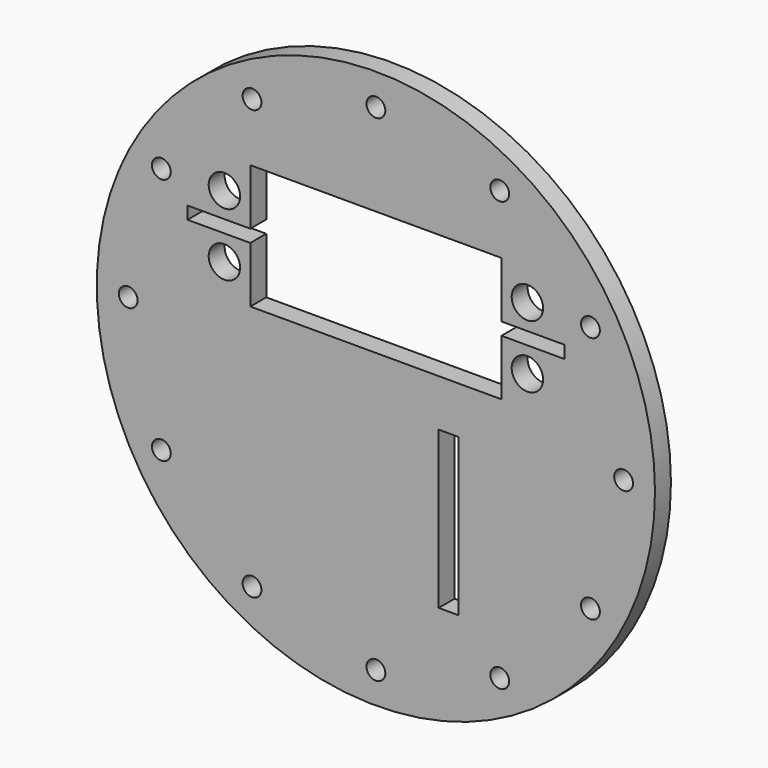
from build123d import *

# Parameters (mm, degrees)
F0_R     = 44.45
F0_R_2   = 1.5
F0_R_3   = 2.5
F1_DEPTH = 3.175


# Not quite as in the source:
# - a length typed as a fraction of an inch, garbled in the dataset ("3 / 203.2 mm" for 3/8 in), is restored


with BuildPart() as f1:
    # F0 (on Front) → F1 (new body)
    with BuildSketch(Plane.XZ):
        Circle(F0_R)
        with Locations((-19.725, -34.1647021793)):
            Circle(F0_R_2, mode=Mode.SUBTRACT)
        with Locations((-34.1647021793, -19.725)):
            Circle(F0_R_2, mode=Mode.SUBTRACT)
        with Locations((0, -39.45)):
            Circle(F0_R_2, mode=Mode.SUBTRACT)
        with Locations((19.725, -34.1647021793)):
            Circle(F0_R_2, mode=Mode.SUBTRACT)
        Polygon((10, -27.5), (10, -15), (10, -2.5), (13.175, -2.5), (13.175, -15), (13.175, -27.5), align=None, mode=Mode.SUBTRACT)
        with Locations((34.1647021793, -19.725)):
            Circle(F0_R_2, mode=Mode.SUBTRACT)
        with Locations((-39.45, 0)):
            Circle(F0_R_2, mode=Mode.SUBTRACT)
        with Locations((-24.125, 9.91)):
            Circle(F0_R_3, mode=Mode.SUBTRACT)
        with Locations((-34.1647021793, 19.725)):
            Circle(F0_R_2, mode=Mode.SUBTRACT)
        with Locations((-24.125, 19.91)):
            Circle(F0_R_3, mode=Mode.SUBTRACT)
        with Locations((-19.725, 34.1647021793)):
            Circle(F0_R_2, mode=Mode.SUBTRACT)
        Polygon((-20, 15.91), (-20, 24.82), (20, 24.82), (20, 15.91), (30, 15.91), (30, 13.91), (20, 13.91), (20, 5), (-20, 5), (-20, 13.91), (-30, 13.91), (-30, 15.91), align=None, mode=Mode.SUBTRACT)
        with Locations((24.125, 9.91)):
            Circle(F0_R_3, mode=Mode.SUBTRACT)
        with Locations((39.45, 0)):
            Circle(F0_R_2, mode=Mode.SUBTRACT)
        with Locations((24.125, 19.91)):
            Circle(F0_R_3, mode=Mode.SUBTRACT)
        with Locations((34.1647021793, 19.725)):
            Circle(F0_R_2, mode=Mode.SUBTRACT)
        with Locations((0, 39.45)):
            Circle(F0_R_2, mode=Mode.SUBTRACT)
        with Locations((19.725, 34.1647021793)):
            Circle(F0_R_2, mode=Mode.SUBTRACT)
    extrude(amount=F1_DEPTH)


solid = f1.part
